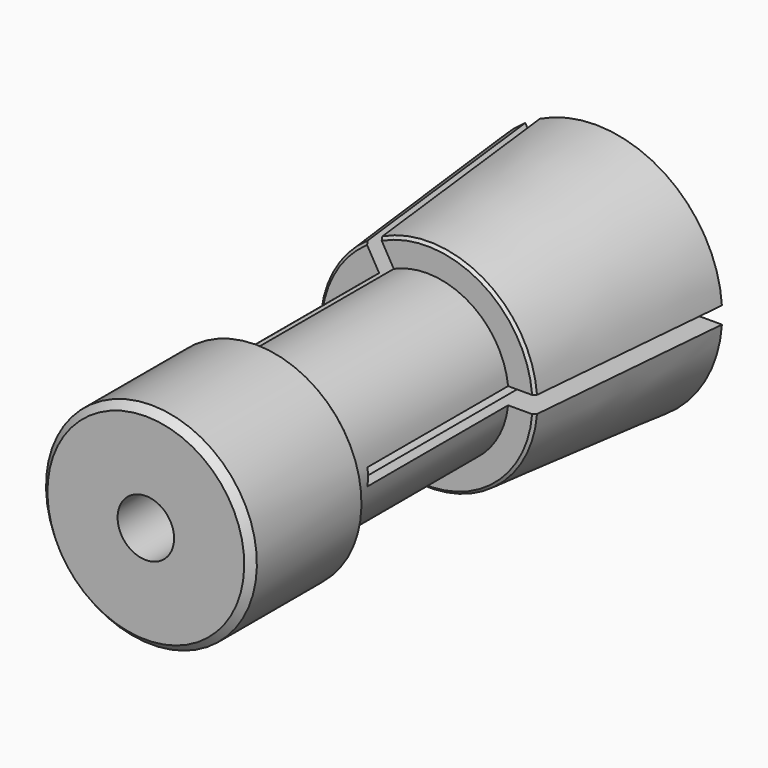
from build123d import *

# Parameters (mm, degrees)
F2_R         = 6.35
F3_DEPTH     = 34.925
F5_D         = 5.1054
F9_DEPTH     = 34.925
F10_SIZE     = 0.635
F11_T4_ANGLE = 118.0970990721
F11_T6_ANGLE = 118.1103265481
F11_T8_ANGLE = 118.1037128101


# Not quite as in the source:
# - a fillet or chamfer that OpenCascade refuses, or shapes differently, is made with other operations: its cross-section is extruded or revolved along the edge and cut away or added


with BuildPart() as f1:
    # F0 (on Right) → F1 (revolve)
    with BuildSketch(Plane.YZ):
        Polygon((-11.3264165741, 23.7704595025), (-40.3521669373, 23.7704595025), (-40.3521669373, 14.2454595025), (10.4478330627, 14.2454595025), (10.4478330627, 25.6754595025), align=None)
    revolve(axis=Axis((0, -14.9521669373, 14.2454595025), (0, 1, 0)))

    # F2 (on face) → F3 (cut)
    with BuildSketch(Plane(origin=(0, 10.4478330627, 0), x_dir=(-1, 0, 0), z_dir=(0, 1, 0))):
        with Locations((0, 14.2454595025)):
            Circle(F2_R)
    extrude(amount=-F3_DEPTH, mode=Mode.SUBTRACT)

    # F5 (through all)
    with Locations(Plane.XZ.offset(40.3521669373)):
        with Locations((0, 14.2454595025)):
            Hole(F5_D / 2)

    # F6 (on Right) → F7 (revolve, cut)
    with BuildSketch(Plane.YZ):
        Polygon((-11.3264165741, 23.7704595025), (-27.6521669373, 23.7704595025), (-27.6521669373, 21.6114595025), (-8.6021669373, 21.6114595025), (-8.6021669373, 24.0088004624), align=None)
    revolve(axis=Axis((0, -14.9521669373, 14.2454595025), (0, 1, 0)), mode=Mode.SUBTRACT)

    # F8 (on face) → F9 (cut)
    with BuildSketch(Plane(origin=(0, 10.4478330627, 0), x_dir=(-1, 0, 0), z_dir=(0, 1, 0))):
        with BuildLine():
            Line((-6.3041142122, 15.0074595025), (-11.4045717149, 15.0074595025))
            ThreePointArc((-11.4045717149, 15.0074595025), (-11.43, 14.2454595025), (-11.4045717149, 13.4834595025))
            Line((-11.4045717149, 13.4834595025), (-6.3041142122, 13.4834595025))
            ThreePointArc((-6.3041142122, 13.4834595025), (-6.35, 14.2454595025), (-6.3041142122, 15.0074595025))
        make_face()
        with BuildLine():
            Line((3.8113822624, 19.3244225118), (6.3611011609, 23.7418426046))
            ThreePointArc((6.3611011609, 23.7418426046), (5.7138574323, 24.1447894416), (5.0411905024, 24.5036902622))
            Line((5.0411905024, 24.5036902622), (2.4914716038, 20.0862701695))
            ThreePointArc((2.4914716038, 20.0862701695), (3.1743652402, 19.7450872465), (3.8113822624, 19.3244225118))
        make_face()
        with BuildLine():
            ThreePointArc((5.04355843, 3.9883927501), (5.7161424915, 4.347448843), (6.3632931846, 4.7505450823))
            Line((6.3632931846, 4.7505450823), (3.8125546144, 9.1673764673))
            ThreePointArc((3.8125546144, 9.1673764673), (3.1756347175, 8.7465646917), (2.4928198598, 8.4052241351))
            Line((2.4928198598, 8.4052241351), (5.04355843, 3.9883927501))
        make_face()
    extrude(amount=-F9_DEPTH, mode=Mode.SUBTRACT)

    # F10
    f10_edges = [f1.edges().sort_by_distance(p)[0] for p in [
        (0, -40.352167, 4.72046),
    ]]
    chamfer(f10_edges, length=F10_SIZE)

    # F11: chamfer of 0.254 on 4 edges, made by hand

    # F11_s1 → F11_t2 (revolve, cut)
    with BuildSketch(Plane.YZ):
        Polygon((-27.9061669373, 23.7704595025), (-27.6521669373, 23.5164595025), (-27.6521669373, 23.7704595025), align=None)
    revolve(axis=Axis((0, -27.6521669373, 14.2454595025), (0, 1, 0)), mode=Mode.SUBTRACT)

    # F11_s3 → F11_t4 (revolve, cut)
    with BuildSketch(Plane(origin=(6.0463708023, 0, 3.3578022312), x_dir=(0, 1, 0), z_dir=(-0.8742366104, 0, -0.485500102))):
        Polygon((-8.6021669373, -21.9844950709), (-8.3703044959, -22.2375285242), (-8.6021669373, -22.2172431891), align=None)
    revolve(axis=Axis((0, -8.6021669373, 14.2454595025), (0, 1, 0)), revolution_arc=F11_T4_ANGLE, mode=Mode.SUBTRACT)

    # F11_s5 → F11_t6 (revolve, cut)
    with BuildSketch(Plane(origin=(0.2356940066, 0, 14.2415588295), x_dir=(0, 1, 0), z_dir=(0.0165474678, 0, 0.9998630813))):
        Polygon((-8.6021669373, -9.2948665597), (-8.3703044959, -9.547900013), (-8.6021669373, -9.5276146779), align=None)
    revolve(axis=Axis((0, -8.6021669373, 14.2454595025), (0, 1, 0)), revolution_arc=F11_T6_ANGLE, mode=Mode.SUBTRACT)

    # F11_s7 → F11_t8 (revolve, cut)
    with BuildSketch(Plane(origin=(-6.2837082468, 0, 3.7688827395), x_dir=(0, 1, 0), z_dir=(0.8575737294, 0, -0.5143610587))):
        Polygon((-8.6021669373, 2.6859389904), (-8.3703044959, 2.4329055371), (-8.6021669373, 2.4531908722), align=None)
    revolve(axis=Axis((0, -8.6021669373, 14.2454595025), (0, 1, 0)), revolution_arc=F11_T8_ANGLE, mode=Mode.SUBTRACT)


solid = f1.part
